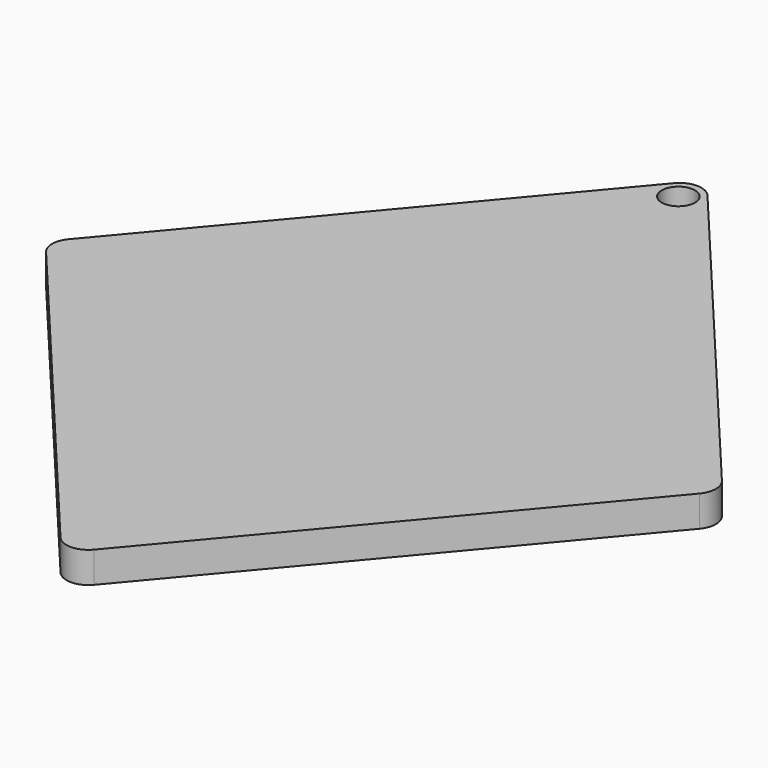
from build123d import *

# Parameters (mm, degrees)
F0_R     = 3.40817912
F1_DEPTH = 6.35


# Not quite as in the source:
# - a length typed as a fraction of an inch, garbled in the dataset ("3 / 203.2 mm" for 3/8 in), is restored


with BuildPart() as f1:
    # F0 (on Top) → F1 (new body)
    with BuildSketch(Plane.XY):
        with BuildLine():
            ThreePointArc((3.4050675497, 78.4919985147), (0, 80.0798075896), (-3.4050675497, 78.4919985147))
            Line((-3.4050675497, 78.4919985147), (-66.8702067023, 2.8571909251))
            ThreePointArc((-66.8702067023, 2.8571909251), (-67.9101391526, 0), (-66.8702067023, -2.8571909251))
            Line((-66.8702067023, -2.8571909251), (-3.4050675497, -78.4919985147))
            ThreePointArc((-3.4050675497, -78.4919985147), (0, -80.0798075896), (3.4050675497, -78.4919985147))
            Line((3.4050675497, -78.4919985147), (66.8702067023, -2.8571909251))
            ThreePointArc((66.8702067023, -2.8571909251), (67.9101391526, 0), (66.8702067023, 2.8571909251))
            Line((66.8702067023, 2.8571909251), (3.4050675497, 78.4919985147))
        make_face()
        with Locations((0, 75.311)):
            Circle(F0_R, mode=Mode.SUBTRACT)
    extrude(amount=F1_DEPTH)


solid = f1.part
